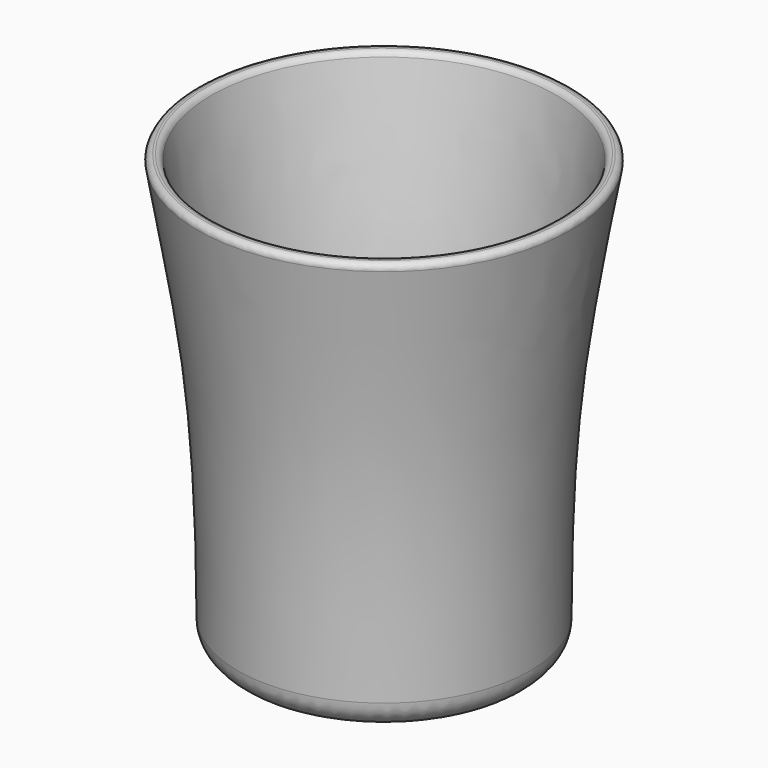
from build123d import *

# Parameters (mm, degrees)
F2_T = -3
F3_R = 6
F4_R = 1.27
F5_R = 2.54


# Not quite as in the source:
# - a feature names something its author has since deleted; it is built from what else it names


with BuildPart() as f1:
    # F0 (on Front) → F1 (revolve)
    with BuildSketch(Plane.XZ):
        with BuildLine():
            Line((0, 0), (32, 0))
            add(Edge.make_bspline(
                [(32, 0), (31.9638415047, 21.1603806981), (33.1788966398, 47.9824141738), (35.859430952, 66.6345209779), (41, 95)],
                knots=[0, 0, 0, 0, 0.4874228368, 1, 1, 1, 1], degree=3))
            Line((41, 95), (0, 95))
            Line((0, 95), (0, 0))
        make_face()
    revolve(axis=Axis((0, 0, 47.5), (0, 0, -1)))

    # F2
    f2_openings = [f1.faces().sort_by_distance(p)[0] for p in [
        (0, 0, 95),
    ]]
    offset(amount=F2_T, openings=f2_openings)

    # F3
    f3_edges = [f1.edges().sort_by_distance(p)[0] for p in [
        (-32, 0, 0),
    ]]
    fillet(f3_edges, radius=F3_R)

    # F4
    f4_edges = [f1.edges().sort_by_distance(p)[0] for p in [
        (-41, 0, 95),
        (-37.951177, 0, 95),
    ]]
    fillet(f4_edges, radius=F4_R)

    # F5
    f5_edges = [f1.edges().sort_by_distance(p)[0] for p in [
        (-28.999113, 0, 3),
    ]]
    fillet(f5_edges, radius=F5_R)


solid = f1.part
